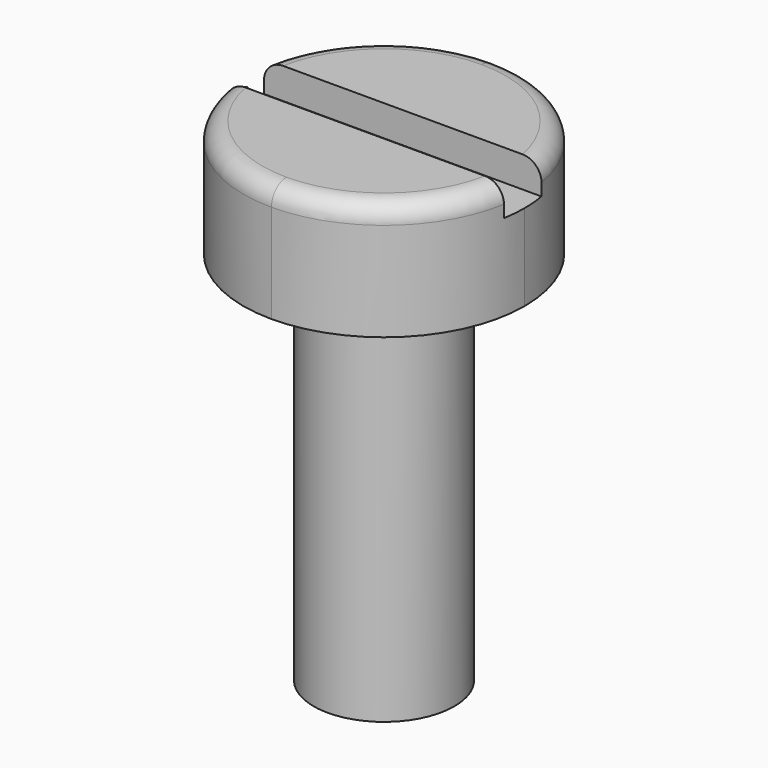
from build123d import *

# Parameters (mm, degrees)
F1_DEPTH    = 3.81
F2_T1_DEPTH = 22.225
F3_R        = 3.80999
F0_W        = 1.905
F0_H        = 10.16
F5_R        = 0.508
F7_DEPTH    = 0.8382


# Not quite as in the source:
# - a fillet or chamfer that OpenCascade refuses, or shapes differently, is made with other operations: its cross-section is extruded or revolved along the edge and cut away or added
# - a fillet or chamfer is up to 0.001 mm smaller than in the source, because OpenCascade refuses the exact size
# - ends of sketch curves that miss each other by under 0.0002 mm in the source are joined
# - a feature names something its author has since deleted; it is built from what else it names


with BuildPart() as f1:
    # F0 (on Front) → F1 (new body, symmetric)
    with BuildSketch(Plane.XZ):
        Polygon((-3.81, 3.175), (-3.81, 0), (-1.905, 0), (0, 0), (1.905, 0), (3.81, 0), (3.81, 3.175), align=None)
    extrude(amount=F1_DEPTH, both=True)

    # F2: fillet of radius 3.81 on 2 edges, made by hand

    # F2_s2 → F2_t1 (cut)
    with BuildSketch(Plane.XY.offset(-9.525)):
        with BuildLine():
            ThreePointArc((-3.81, 0), (-2.6940768363, -2.6940768363), (0, -3.81))
            Line((0, -3.81), (-3.81, -3.81))
            Line((-3.81, -3.81), (-3.81, 0))
        make_face()
        with BuildLine():
            ThreePointArc((-3.81, 0), (-2.6940768363, 2.6940768363), (0, 3.81))
            Line((0, 3.81), (-3.81, 3.81))
            Line((-3.81, 3.81), (-3.81, 0))
        make_face()
    extrude(amount=F2_T1_DEPTH, mode=Mode.SUBTRACT)

    # F3 (radius 3.81 in the source; OpenCascade refuses exactly that, so slightly less here)
    f3_edges = [f1.edges().sort_by_distance(p)[0] for p in [
        (3.81, -3.81, 1.5875),
        (3.81, 3.81, 1.5875),
    ]]
    fillet(f3_edges, radius=F3_R)

    # F0 (on Front) → F4 (revolve)
    with BuildSketch(Plane.XZ):
        with Locations((0.9525, -5.08)):
            Rectangle(F0_W, F0_H)
    revolve(axis=Axis((0, 0, -5.08), (0, 0, 1)))

    # F5
    f5_edges = [f1.edges().sort_by_distance(p)[0] for p in [
        (-2.694077, -2.694077, 3.175),
        (2.69408, -2.69408, 3.175),
        (5e-06, -3.81, 3.175),
        (-2.694077, 2.694077, 3.175),
        (2.69408, 2.69408, 3.175),
        (5e-06, 3.81, 3.175),
    ]]
    fillet(f5_edges, radius=F5_R)

    # F6 (on face) → F7 (cut)
    with BuildSketch(Plane.XY.offset(3.175)):
        with BuildLine():
            Line((-3.2403671088, 0.635), (-3.8071805373, 0.635))
            Line((-3.8071805373, 0.635), (-3.8071805373, -0.635))
            Line((-3.8071805373, -0.635), (-3.2403671088, -0.635))
            ThreePointArc((-3.2403671088, -0.635), (-3.2865556585, -0.3189920114), (-3.302, 0))
            ThreePointArc((-3.302, 0), (-3.2865556585, 0.3189920114), (-3.2403671088, 0.635))
        make_face()
        with BuildLine():
            Line((3.2403688783, 0.635), (-3.2403671088, 0.635))
            ThreePointArc((-3.2403671088, 0.635), (-3.2865556585, 0.3189920114), (-3.302, 0))
            ThreePointArc((-3.302, 0), (-3.2865556585, -0.3189920114), (-3.2403671088, -0.635))
            Line((-3.2403671088, -0.635), (3.2403688783, -0.635))
            ThreePointArc((3.2403688783, -0.635), (3.2865561029, -0.3189969493), (3.302, -1e-05))
            ThreePointArc((3.302, -1e-05), (3.2865561029, 0.3189969493), (3.2403688783, 0.635))
        make_face()
        with BuildLine():
            Line((3.8128194627, 0.635), (3.2403688783, 0.635))
            ThreePointArc((3.2403688783, 0.635), (3.2865561029, 0.3189969493), (3.302, 1e-05))
            ThreePointArc((3.302, 1e-05), (3.2865561029, -0.3189969493), (3.2403688783, -0.635))
            Line((3.2403688783, -0.635), (3.8128194627, -0.635))
            Line((3.8128194627, -0.635), (3.8128194627, 0.635))
        make_face()
    extrude(amount=-F7_DEPTH, mode=Mode.SUBTRACT)


solid = f1.part
